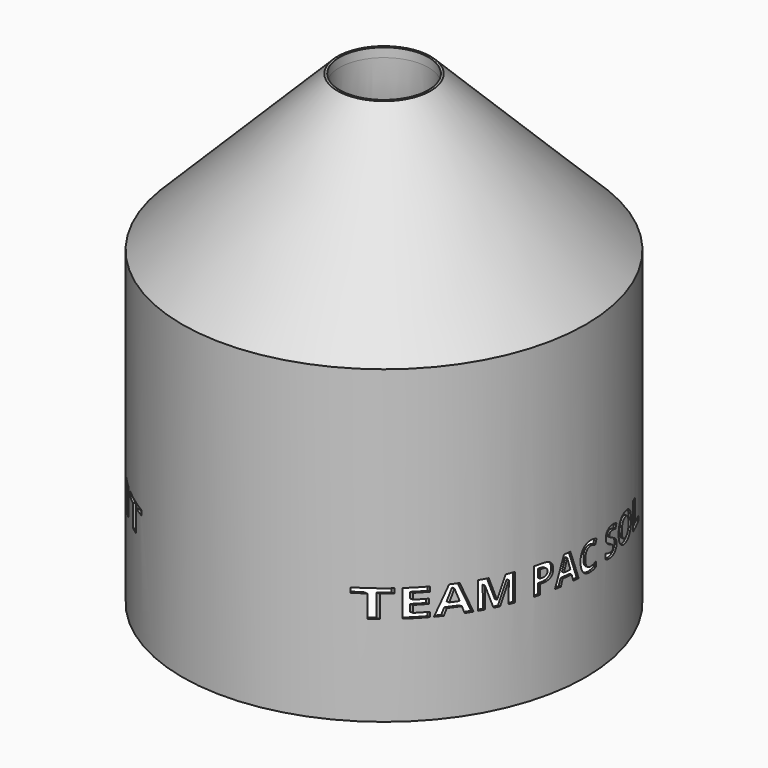
from build123d import *

# Parameters (mm, degrees)
F0_R         = 330.3018032
F1_DEPTH     = 762
F3_SIZE      = 254
F4_R         = 72.719663095
F5_DEPTH     = 762.001
F6_R         = 326.9239246311
F7_DEPTH     = 406.4
F9_TEXT_SIZE = 61.9637055529
F10_DEPTH    = 381


# Not quite as in the source:
# - a fillet or chamfer that OpenCascade refuses, or shapes differently, is made with other operations: its cross-section is extruded or revolved along the edge and cut away or added
# - Text() gives the source's letters only with a copy of the font that has no kerning and outlines rounded to 1/6400 em; it was checked with that copy


with BuildPart() as f1:
    # F0 (on Top) → F1 (new body)
    with BuildSketch(Plane.XY):
        Circle(F0_R)
    extrude(amount=F1_DEPTH)

    # F3
    f3_edges = [f1.edges().sort_by_distance(p)[0] for p in [
        (-330.301803, 0, 762),
    ]]
    chamfer(f3_edges, length=F3_SIZE)

    # F4 (on face) → F5 (cut, through all)
    with BuildSketch(Plane.XY.offset(762)):
        Circle(F4_R)
    extrude(amount=-F5_DEPTH, mode=Mode.SUBTRACT)

    # F6 (on face) → F7 (cut)
    with BuildSketch(Plane(origin=(0, 0, 0), x_dir=(1, 0, 0), z_dir=(0, 0, -1))):
        Circle(F6_R)
    extrude(amount=-F7_DEPTH, mode=Mode.SUBTRACT)

    # F8: fillet of radius 355.6 on 1 edges, made by hand

    # F8_s1 → F8_t2 (revolve, cut)
    with BuildSketch(Plane.XZ):
        with BuildLine():
            ThreePointArc((72.719663095, 747.2375921482), (143.2690670618, 534.6405138495), (326.9239246311, 406.4))
            Line((326.9239246311, 406.4), (324.8960098618, 399.583248157))
            ThreePointArc((324.8960098618, 399.583248157), (199.8217938631, 399.288), (72.719663095, 399.288))
            Line((72.719663095, 399.288), (65.607663095, 406.4))
            Line((65.607663095, 406.4), (65.607663095, 747.2375921482))
            Line((65.607663095, 747.2375921482), (72.719663095, 747.2375921482))
        make_face()
    revolve(axis=Axis((0, 0, 406.4), (0, 0, 1)), mode=Mode.SUBTRACT)

    # F9 (on Right) → F10 (cut, symmetric)
    with BuildSketch(Plane.YZ):
        with Locations((-283.9064598083, 148.2212990522)):
            Text('TEAM PAC SOL', F9_TEXT_SIZE, font='Open Sans', font_style=FontStyle.BOLD, text_align=(TextAlign.LEFT, TextAlign.BOTTOM))
    extrude(amount=F10_DEPTH, both=True, mode=Mode.SUBTRACT)


solid = f1.part
